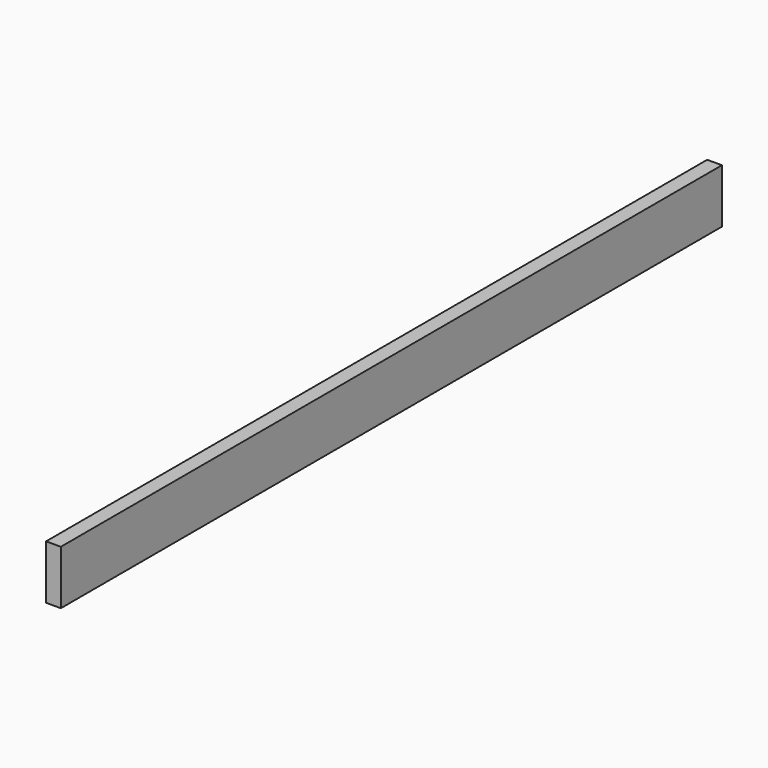
from build123d import *

# Parameters (mm, degrees)
F1_W     = 38.1
F1_H     = 139.7
F2_DEPTH = 2133.6


# Not quite as in the source:
# - a variable given as a bare number and used for a length is read in inches; the dataset says mm whatever the document's units were


with BuildPart() as f2:
    # F1 (on Front) → F2 (new body)
    with BuildSketch(Plane.XZ):
        with Locations((-151.3417023118, 69.85)):
            Rectangle(F1_W, F1_H)
    extrude(amount=F2_DEPTH)


solid = f2.part
